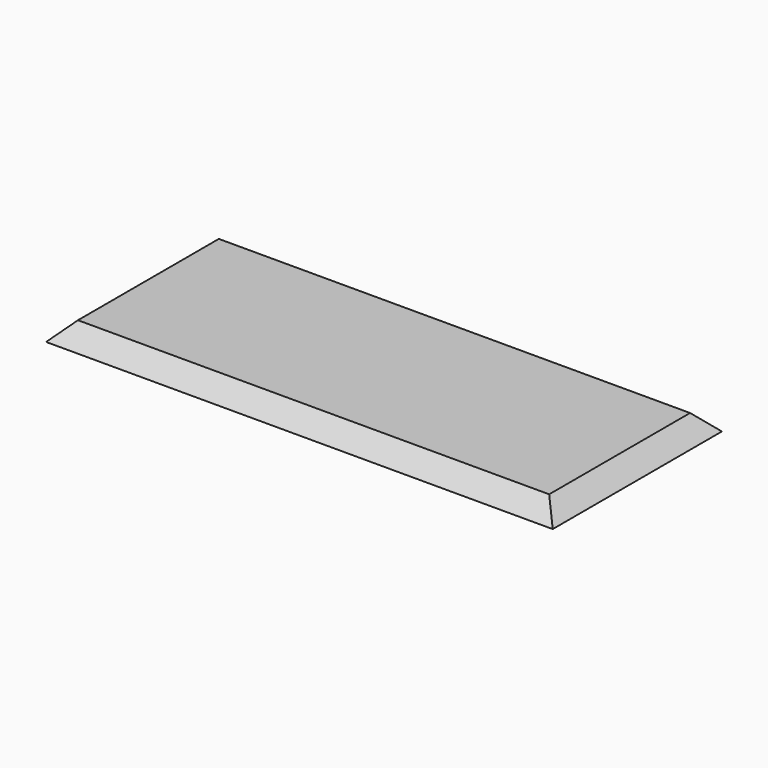
from build123d import *

# Parameters (mm, degrees)
F0_W     = 630
F0_H     = 263
F1_DEPTH = 22
F2_SIZE  = 21.99999


# Not quite as in the source:
# - a fillet or chamfer is up to 0.001 mm smaller than in the source, because OpenCascade refuses the exact size


with BuildPart() as f1:
    # F0 (on Top) → F1 (new body)
    with BuildSketch(Plane.XY):
        Rectangle(F0_W, F0_H)
    extrude(amount=F1_DEPTH)

    # F2 (size 22 in the source; OpenCascade refuses exactly that, so slightly less here)
    f2_edges = [f1.edges().sort_by_distance(p)[0] for p in [
        (-315, 0, 22),
        (0, 131.5, 22),
        (0, -131.5, 22),
        (315, 0, 22),
    ]]
    chamfer(f2_edges, length=F2_SIZE)


solid = f1.part
